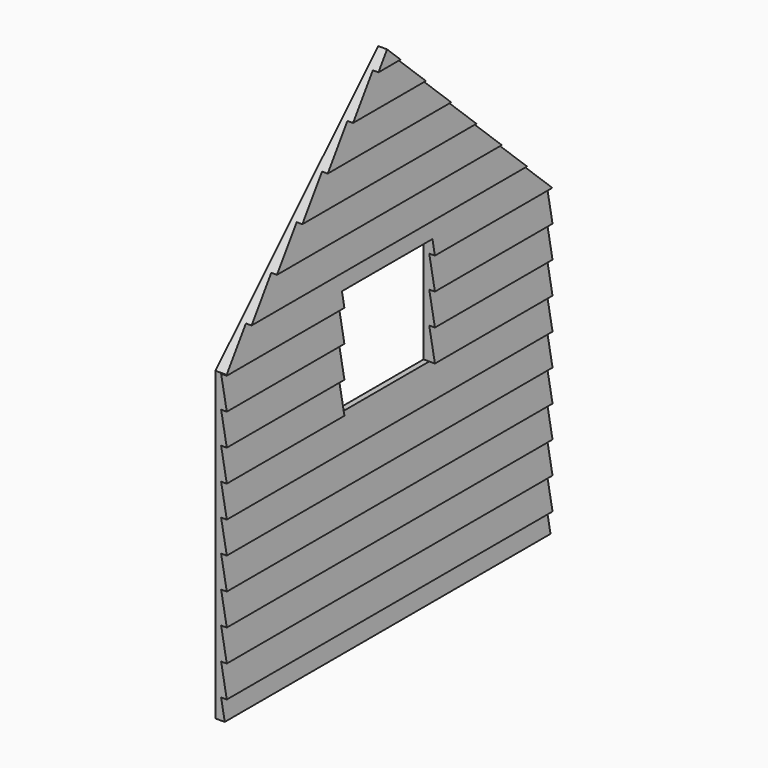
from build123d import *

# Parameters (mm, degrees)
F1_DEPTH = 0.5
F3_DEPTH = 36
F4_DEPTH = 36
F5_DEPTH = 25
F7_DEPTH = 25
F8_DEPTH = 0.223


with BuildPart() as f1:
    # F0 (on Right) → F1 (new body)
    with BuildSketch(Plane.YZ):
        Polygon((-35.463306278, 10.7429168718), (-71.463306278, 10.7429168718), (-71.463306278, 8.9429168718), (-70.463306278, 8.9429168718), (-36.463306278, 8.9429168718), (-35.463306278, 8.9429168718), align=None)
    extrude(amount=F1_DEPTH)

    # F2 (on face) → F3 (join)
    with BuildSketch(Plane.XZ.offset(71.463306278)):
        Polygon((0.5, 8.9429168718), (0.8214285714, 8.9429168718), (0.5, 10.7429168718), align=None)
    extrude(amount=-F3_DEPTH)

    # F2 (on face) → F4 (join)
    with BuildSketch(Plane.XZ.offset(71.463306278)):
        Polygon((0, 10.7429168718), (0.5, 10.7429168718), (1, 10.7429168718), (0.5, 13.5429168718), (1, 13.5429168718), (0.5, 16.3429168718), (1, 16.3429168718), (0.5, 19.1429168718), (1, 19.1429168718), (0.5, 21.9429168718), (1, 21.9429168718), (0.5, 24.7429168718), (1, 24.7429168718), (0.5, 27.5429168718), (1, 27.5429168718), (0.5, 30.3429168718), (1, 30.3429168718), (0.5, 33.1429168718), (1, 33.1429168718), (0.5, 35.9429168718), (1, 35.9429168718), (0.5, 38.7429168718), (1, 38.7429168718), (0.5, 41.5429168718), (1, 41.5429168718), (0.5, 44.3429168718), (1, 44.3429168718), (0.5, 47.1429168718), (1, 47.1429168718), (0.5, 49.9429168718), (1, 49.9429168718), (0.5, 52.7429168718), (1, 52.7429168718), (0.6579817238, 54.6582192183), (0.5, 54.6582192183), (0, 54.6582192183), align=None)
    extrude(amount=-F4_DEPTH)

    # F0 (on Right) → F5 (cut)
    with BuildSketch(Plane.YZ):
        Polygon((-58.463306278, 36.9429168718), (-58.463306278, 35.9429168718), (-58.463306278, 33.1429168718), (-58.463306278, 30.3429168718), (-58.463306278, 27.5429168718), (-48.463306278, 27.5429168718), (-48.463306278, 30.3429168718), (-48.463306278, 33.1429168718), (-48.463306278, 35.9429168718), (-48.463306278, 36.9429168718), (-57.463306278, 36.9429168718), align=None)
    extrude(amount=F5_DEPTH, mode=Mode.SUBTRACT)

    # F6 (on face) → F7 (cut)
    with BuildSketch(Plane(origin=(0, 0, 0), x_dir=(0, -1, 0), z_dir=(-1, 0, 0))):
        Polygon((35.463306278, 54.6582192183), (35.463306278, 35.9216630459), (53.4756928682, 53.9652556181), (71.463306278, 36.0087513756), (71.463306278, 54.6582192183), align=None)
    extrude(amount=-F7_DEPTH, mode=Mode.SUBTRACT)

    # F8 (cut): a face of the model
    f8_faces = [f1.faces().sort_by_distance(p)[0] for p in [
        (0.4107142857, -53.463306278, 36.9429168718),
    ]]
    extrude(f8_faces, amount=-F8_DEPTH, mode=Mode.SUBTRACT)


solid = f1.part
